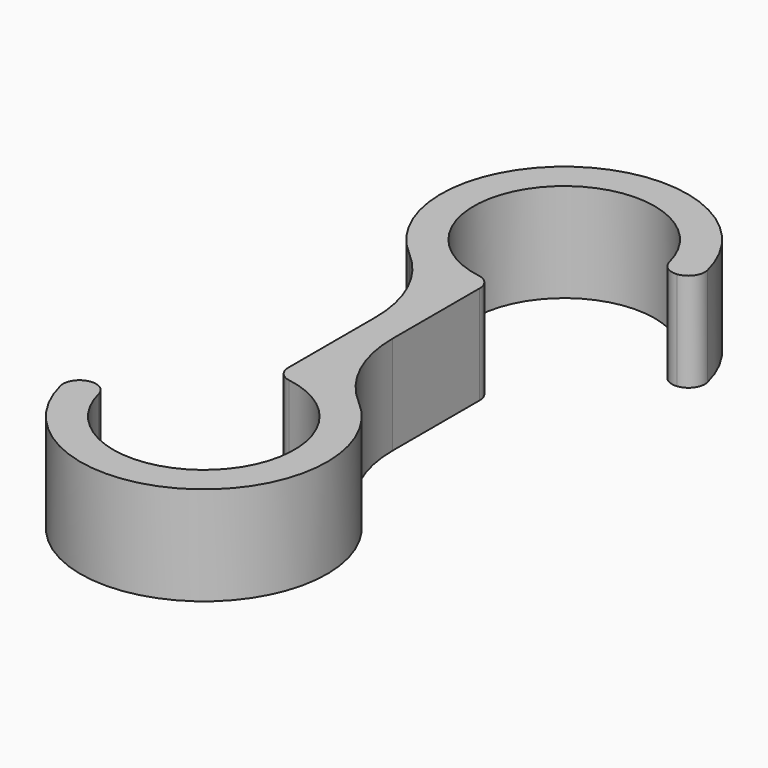
from build123d import *

# Parameters (mm, degrees)
F1_DEPTH = 7.62
F2_R     = 10.16
F3_R     = 1.26999


# Not quite as in the source:
# - a fillet or chamfer is up to 0.001 mm smaller than in the source, because OpenCascade refuses the exact size


with BuildPart() as f1:
    # F0 (on Top) → F1 (new body)
    with BuildSketch(Plane.XY):
        with BuildLine():
            ThreePointArc((0, -6.985), (-5.1498821976, 4.7189976002), (6.9584199662, 0.6087828631))
            Line((6.9584199662, 0.6087828631), (9.4887544993, 0.8301584497))
            ThreePointArc((9.4887544993, 0.8301584497), (-6.0928284325, 7.3214115232), (-2.54, -9.1800885072))
            Line((-2.54, -9.1800885072), (-2.54, -22.0943992214))
            Line((-2.54, -22.0943992214), (-2.54, -24.6343992214))
            ThreePointArc((-2.54, -24.6343992214), (2.6098821976, -36.3383968216), (-9.4984199662, -32.2281820845))
            Line((-9.4984199662, -32.2281820845), (-12.0287544993, -32.4495576711))
            ThreePointArc((-12.0287544993, -32.4495576711), (3.5528284325, -38.9408107447), (0, -22.4393107142))
            Line((0, -22.4393107142), (0, -9.525))
            Line((0, -9.525), (0, -6.985))
        make_face()
    extrude(amount=F1_DEPTH)

    # F2
    f2_edges = [f1.edges().sort_by_distance(p)[0] for p in [
        (-2.54, -9.180089, 3.81),
        (0, -22.439311, 3.81),
    ]]
    fillet(f2_edges, radius=F2_R)

    # F3 (radius 1.27 in the source; OpenCascade refuses exactly that, so slightly less here)
    f3_edges = [f1.edges().sort_by_distance(p)[0] for p in [
        (6.95842, 0.608783, 3.81),
        (9.488754, 0.830158, 3.81),
        (-12.028754, -32.449558, 3.81),
        (-9.49842, -32.228182, 3.81),
        (-2.54, -24.634399, 3.81),
        (0, -6.985, 3.81),
    ]]
    fillet(f3_edges, radius=F3_R)


solid = f1.part
